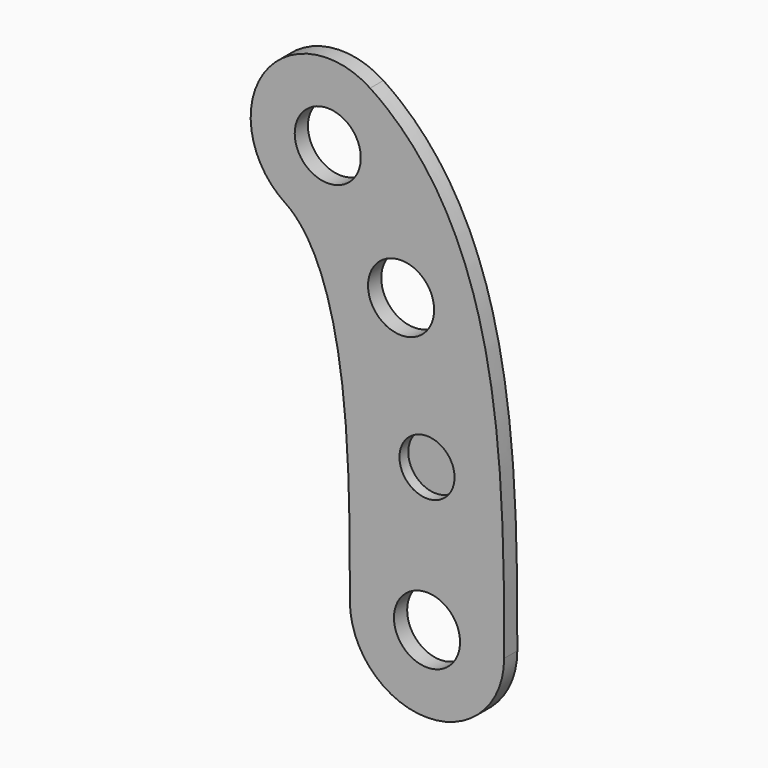
from build123d import *

# Parameters (mm, degrees)
F0_R     = 6
F1_DEPTH = 3
F3_R     = 5.5
F4_DEPTH = 2
F5_R     = 5
F6_DEPTH = 2
F9_ANGLE = 180


# Not quite as in the source:
# - ends of sketch curves that miss each other by under 0.0002 mm in the source are joined
# - the dataset's text gives a spline's control points without its knots; the knots are read off the source's solid


with BuildPart() as f1:
    # F0 (on Front) → F1 (new body)
    with BuildSketch(Plane.XZ):
        with BuildLine():
            add(Edge.make_bspline(
                [(-14, -26), (-14, -22.75), (-14.0004523743, -15.9105291262), (-13.7828666825, -5.0097493319), (-13.1111411806, 6.2097947293), (-11.720563989, 17.4707102353), (-9.6943656003, 26.7000282147), (-7.3231272908, 33.8894297819), (-5.0899646489, 39.15233442), (-2.3107556278, 44.2379137207), (1.1152604329, 49.0651401417), (5.2757801793, 53.5029660938), (8.5623848122, 56.0788774956), (10.3247279458, 57.2378033443)],
                knots=[0, 0, 0, 0, 0.125, 0.25, 0.375, 0.5, 0.625, 0.6875, 0.75, 0.8125, 0.875, 0.9375, 1, 1, 1, 1], degree=3))
            ThreePointArc((-14, -26), (0, -40), (14, -26))
            add(Edge.make_bspline(
                [(14, -26), (14, -22.75), (14.0004523743, -16.1086995406), (14.205139987, -6.0382727532), (14.8002343988, 3.7711749321), (15.9432970346, 12.9047719201), (17.4360428506, 19.5652612944), (18.9356431663, 24.0782015665), (20.186235287, 27.0007682339), (21.5241909854, 29.4228421126), (22.9015337641, 31.3389176928), (24.2833500376, 32.7935083509), (25.2194773121, 33.5209300274), (25.7092571932, 33.8430120472)],
                knots=[0, 0, 0, 0, 0.125, 0.25, 0.375, 0.5, 0.625, 0.6875, 0.75, 0.8125, 0.875, 0.9375, 0.9999998504, 0.9999998504, 0.9999998504, 0.9999998504], degree=3))
            ThreePointArc((25.7092571932, 33.8430120472), (29.7143803557, 53.2326803132), (10.3247279458, 57.2378033443))
        make_face()
        with Locations((0, -26)):
            Circle(F0_R, mode=Mode.SUBTRACT)
        with Locations((4.704827633, 25.5707762288)):
            Circle(F0_R, mode=Mode.SUBTRACT)
        with Locations((18.0169899591, 45.5404115335)):
            Circle(F0_R, mode=Mode.SUBTRACT)
    extrude(amount=F1_DEPTH)


with BuildPart() as f2_1:
    # F2: copy of F1
    add(f1.part.moved(Location((50.8967, 0, 0))))

    # F3 (on face) → F4 (cut)
    with BuildSketch(Plane.XZ.offset(3)):
        with Locations((50.8965918246, 0)):
            Circle(F3_R)
    extrude(amount=-F4_DEPTH, mode=Mode.SUBTRACT)


with BuildPart() as f1_1:
    add(f1.part)

    # F5 (on face) → F6 (cut)
    with BuildSketch(Plane(origin=(0, 0, 0), x_dir=(-1, 0, 0), z_dir=(0, 1, 0))):
        Circle(F5_R)
    extrude(amount=-F6_DEPTH, mode=Mode.SUBTRACT)


with BuildPart() as f1_2:
    # F9: moved
    add(f1_1.part.rotate(Axis((0, 0, 5.4726116359), (0, 0, -1)), F9_ANGLE))


solid = f1_2.part
